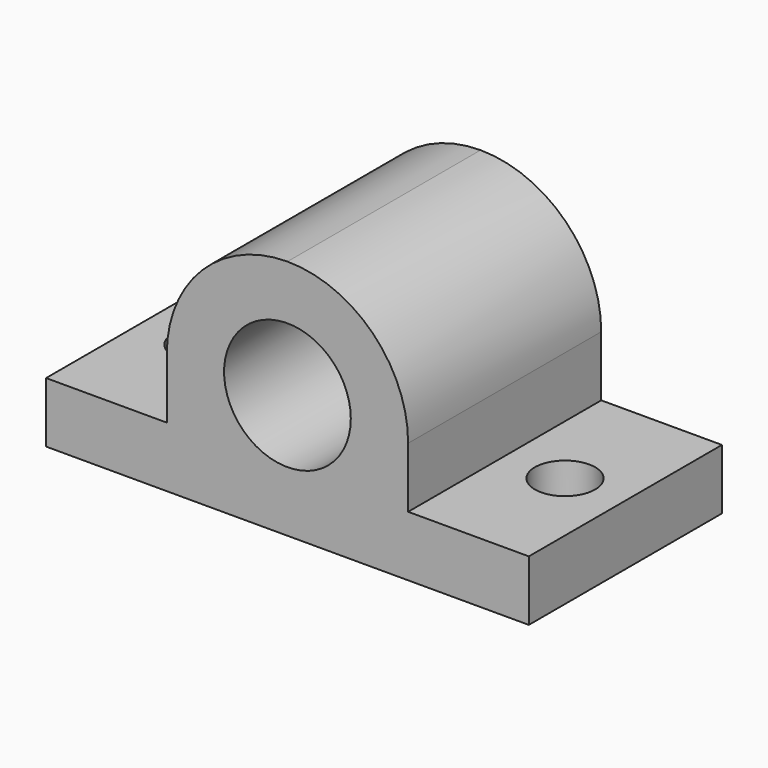
from build123d import *

# Parameters (mm, degrees)
F0_W     = 40
F0_H     = 20
F0_R     = 2.5
F1_DEPTH = 5
F2_W     = 20
F2_H     = 20
F3_DEPTH = 15
F4_R     = 5.25
F5_DEPTH = 25
F6_R     = 9.99999


# Not quite as in the source:
# - a fillet or chamfer is up to 0.001 mm smaller than in the source, because OpenCascade refuses the exact size


with BuildPart() as f1:
    # F0 (on Top) → F1 (new body)
    with BuildSketch(Plane.XY):
        Rectangle(F0_W, F0_H)
        with Locations((-15, 0)):
            Circle(F0_R, mode=Mode.SUBTRACT)
        with Locations((15, 0)):
            Circle(F0_R, mode=Mode.SUBTRACT)
    extrude(amount=F1_DEPTH)

    # F2 (on face) → F3 (join)
    with BuildSketch(Plane.XY.offset(5)):
        Rectangle(F2_W, F2_H)
    extrude(amount=F3_DEPTH)

    # F4 (on face) → F5 (cut)
    with BuildSketch(Plane.XZ.offset(10)):
        with Locations((0, 10.25)):
            Circle(F4_R)
    extrude(amount=-F5_DEPTH, mode=Mode.SUBTRACT)

    # F6 (radius 10 in the source; OpenCascade refuses exactly that, so slightly less here)
    f6_edges = [f1.edges().sort_by_distance(p)[0] for p in [
        (-10, 0, 20),
        (10, 0, 20),
    ]]
    fillet(f6_edges, radius=F6_R)


solid = f1.part
